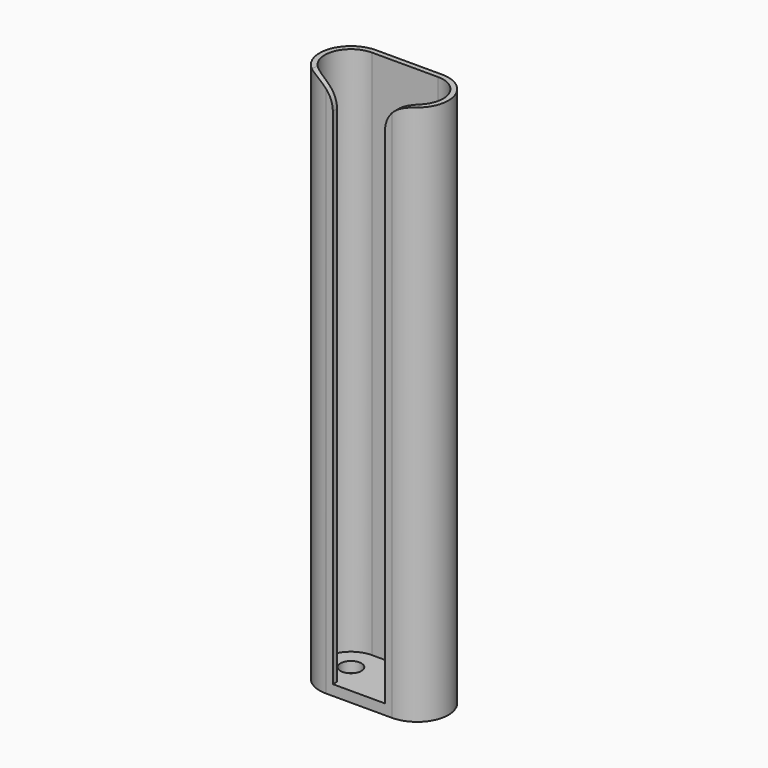
from build123d import *

# Parameters (mm, degrees)
F1_DEPTH       = 304.8
F2_T1_DEPTH    = 33.0000735539
F4_D           = 3
F4_CBORE_D     = 10
F4_CBORE_DEPTH = 1
F5_R           = 6
F6_DEPTH       = 6


# Not quite as in the source:
# - a fillet or chamfer that OpenCascade refuses, or shapes differently, is made with other operations: its cross-section is extruded or revolved along the edge and cut away or added


with BuildPart() as f1:
    # F0 (on Top) → F1 (new body)
    with BuildSketch(Plane.XY):
        with BuildLine():
            ThreePointArc((-19.0469745753, -14.9999264461), (-33.9999816115, 0.0234873165), (-19, 15))
            Line((-19, 15), (0, 15))
            Line((0, 15), (19, 15))
            ThreePointArc((19, 15), (33.9999816115, 0.0234873165), (19.0469745753, -14.9999264461))
            ThreePointArc((19.0469745753, -14.9999264461), (19, -15), (18.9530254247, -14.9999264461))
            Line((18.9530254247, -14.9999264461), (15, -14.9999264461))
            Line((15, -14.9999264461), (15, -18))
            Line((15, -18), (19, -18))
            ThreePointArc((19, -18), (37, 0), (19, 18))
            Line((19, 18), (0, 18))
            Line((0, 18), (-19, 18))
            ThreePointArc((-19, 18), (-37, 0), (-19, -18))
            Line((-19, -18), (-15, -18))
            Line((-15, -18), (-15, -14.9999264461))
            Line((-15, -14.9999264461), (-18.9530254247, -14.9999264461))
            ThreePointArc((-18.9530254247, -14.9999264461), (-19, -15), (-19.0469745753, -14.9999264461))
        make_face()
    extrude(amount=F1_DEPTH)

    # F2: fillet of radius 15 on 2 edges, made by hand

    # F2_s2 → F2_t1 (cut)
    with BuildSketch(Plane.XZ.offset(-7.35539e-05)):
        with BuildLine():
            ThreePointArc((-30, 304.8), (-19.3933982822, 300.4066017178), (-15, 289.8))
            Line((-15, 289.8), (-14.7, 289.8))
            Line((-14.7, 289.8), (-14.7, 305.1))
            Line((-14.7, 305.1), (-30, 305.1))
            Line((-30, 305.1), (-30, 304.8))
        make_face()
        with BuildLine():
            ThreePointArc((30, 304.8), (19.3933982822, 300.4066017178), (15, 289.8))
            Line((15, 289.8), (14.7, 289.8))
            Line((14.7, 289.8), (14.7, 305.1))
            Line((14.7, 305.1), (30, 305.1))
            Line((30, 305.1), (30, 304.8))
        make_face()
    extrude(amount=F2_T1_DEPTH, mode=Mode.SUBTRACT)

    # F4 (through all)
    with Locations(Plane.XZ.offset(-15)):
        with Locations((0, 254.8), (0, 50)):
            CounterBoreHole(F4_D / 2, F4_CBORE_D / 2, F4_CBORE_DEPTH)

    # F5 (on face) → F6 (join)
    with BuildSketch(Plane(origin=(0, 0, 0), x_dir=(1, 0, 0), z_dir=(0, 0, -1))):
        with BuildLine():
            ThreePointArc((-19, 18), (-37, 0), (-19, -18))
            Line((-19, -18), (19, -18))
            ThreePointArc((19, -18), (37, 0), (19, 18))
            Line((19, 18), (-19, 18))
        make_face()
        with Locations((-19, 0)):
            Circle(F5_R, mode=Mode.SUBTRACT)
        with Locations((19, 0)):
            Circle(F5_R, mode=Mode.SUBTRACT)
    extrude(amount=F6_DEPTH)


solid = f1.part
